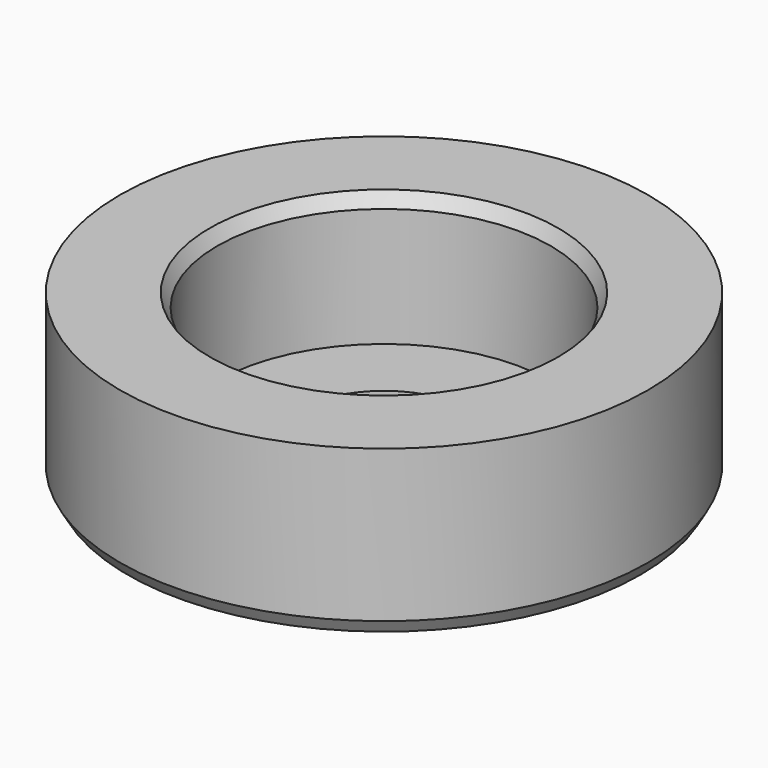
from build123d import *

# Parameters (mm, degrees)
F0_R        = 5.05
F0_R_2      = 2.65
F1_DEPTH    = 1
F0_R_3      = 8
F2_DEPTH    = 5
F3_C1_SIZE2 = 0.4
F3_C1_SIZE  = 0.2309401077
F3_C2_SIZE2 = 0.4
F3_C2_SIZE  = 0.2309401077
F3_C3_SIZE2 = 0.4
F3_C3_SIZE  = 0.2309401077


with BuildPart() as f1:
    # F0 (on Top) → F1 (new body)
    with BuildSketch(Plane.XY):
        Circle(F0_R)
        Circle(F0_R_2, mode=Mode.SUBTRACT)
    extrude(amount=F1_DEPTH)

    # F0 (on Top) → F2 (join)
    with BuildSketch(Plane.XY):
        Circle(F0_R_3)
        Circle(F0_R, mode=Mode.SUBTRACT)
    extrude(amount=F2_DEPTH)

    # F3: chamfer of 0.4 x 0.2309401077 on 3 edges, made by hand

    # F3_c1
    f3_c1_edges = [f1.edges().sort_by_distance(p)[0] for p in [
        (-2.65, 0, 0),
    ]]
    f3_c1_side = f1.faces().sort_by_distance((-2.65, 0, 0.0046188022))[0]
    chamfer(f3_c1_edges, length=F3_C1_SIZE, length2=F3_C1_SIZE2, reference=f3_c1_side)

    # F3_c2
    f3_c2_edges = [f1.edges().sort_by_distance(p)[0] for p in [
        (-8, 0, 0),
    ]]
    f3_c2_side = f1.faces().sort_by_distance((-7.9953811978, 0, 0))[0]
    chamfer(f3_c2_edges, length=F3_C2_SIZE, length2=F3_C2_SIZE2, reference=f3_c2_side)

    # F3_c3
    f3_c3_edges = [f1.edges().sort_by_distance(p)[0] for p in [
        (-5.05, 0, 5),
    ]]
    f3_c3_side = f1.faces().sort_by_distance((-5.0546188022, 0, 5))[0]
    chamfer(f3_c3_edges, length=F3_C3_SIZE, length2=F3_C3_SIZE2, reference=f3_c3_side)


solid = f1.part
